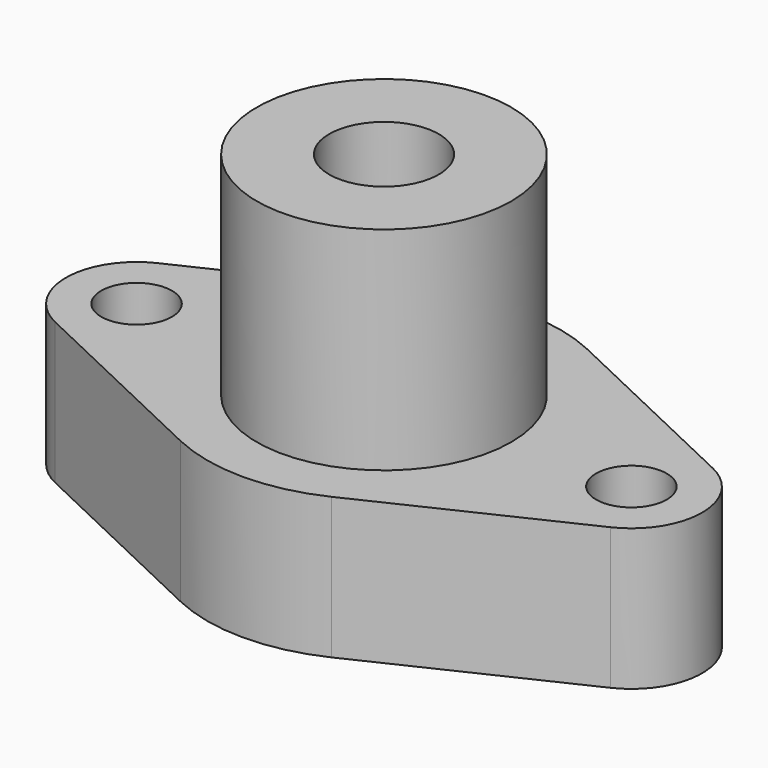
from build123d import *

# Parameters (mm, degrees)
F1_DEPTH = 20
F3_D     = 10
F3_DEPTH = 20
F3_TIP   = 3.0043030951
F4_R     = 18
F5_DEPTH = 30
F7_D     = 15.5
F7_DEPTH = 25
F7_TIP   = 4.6566697975


# Not quite as in the source:
# - ends of sketch curves that miss each other by under 0.0002 mm in the source are joined


with BuildPart() as f1:
    # F0 (on Top) → F1 (new body)
    with BuildSketch(Plane.XY):
        with BuildLine():
            Line((-10.7142857143, 22.5876975726), (-39.2857142857, 9.0350790291))
            ThreePointArc((-39.2857142857, 9.0350790291), (-45, 0), (-39.2857142857, -9.0350790291))
            Line((-39.2857142857, -9.0350790291), (-10.7742508272, -22.5592536221))
            Line((-10.7742508272, -22.5592536221), (-10.7142857143, -22.5876975726))
            ThreePointArc((-10.7142857143, -22.5876975726), (-0.0331846382, -25.000066073), (10.6543206014, -22.6161415232))
            Line((10.6543206014, -22.6161415232), (39.2857142857, -9.0350790291))
            ThreePointArc((39.2857142857, -9.0350790291), (45, 0), (39.2857142857, 9.0350790291))
            Line((39.2857142857, 9.0350790291), (10.7142857143, 22.5876975726))
            ThreePointArc((10.7142857143, 22.5876975726), (0, 25), (-10.7142857143, 22.5876975726))
        make_face()
    extrude(amount=F1_DEPTH)

    # F3
    with Locations(Plane.XY.offset(20)):
        with Locations((-35, 0), (35, 0)):
            Hole(F3_D / 2, depth=F3_DEPTH)
            with Locations((0, 0, -(F3_DEPTH + F3_TIP / 2))):  # 118° drill point
                Cone(0, F3_D / 2, F3_TIP, mode=Mode.SUBTRACT)

    # F4 (on face) → F5 (join)
    with BuildSketch(Plane.XY.offset(20)):
        Circle(F4_R)
    extrude(amount=F5_DEPTH)

    # F7
    with Locations(Plane.XY.offset(50)):
        with Locations((0, 0)):
            Hole(F7_D / 2, depth=F7_DEPTH)
            with Locations((0, 0, -(F7_DEPTH + F7_TIP / 2))):  # 118° drill point
                Cone(0, F7_D / 2, F7_TIP, mode=Mode.SUBTRACT)


solid = f1.part
